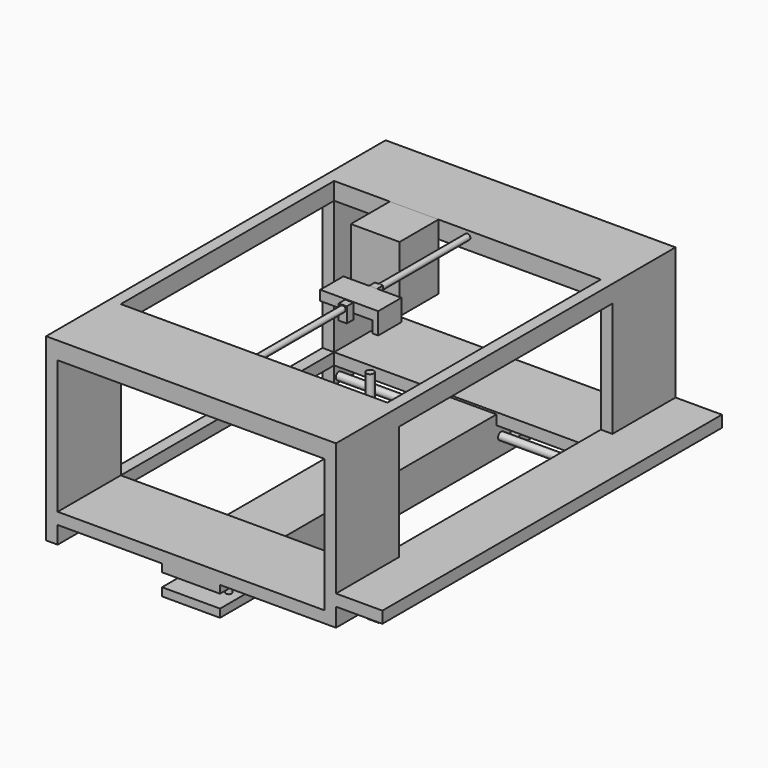
from build123d import *

# Parameters (mm, degrees)
F0_W         = 250
F0_H         = 250
F1_DEPTH     = 70
F2_T         = -10
F3_W         = 230
F3_H         = 120
F4_DEPTH     = 300
F5_W         = 230
F5_H         = 120
F6_DEPTH     = 300
F7_W         = 230
F7_H         = 230
F8_DEPTH     = 500
F9_W         = 10
F9_H         = 10
F1_FACE3_W   = 250
F1_FACE3_H   = 250
F1_FACE3_W_2 = 230
F1_FACE3_H_2 = 230
F10_DEPTH    = 15
F11_R        = 2.5
F12_DEPTH    = 250
F13_W        = 50
F13_H        = 18.5
F14_DEPTH    = 12.5
F16_DEPTH    = 10
F17_W        = 7
F17_H        = 13
F18_DEPTH    = 3.5
F19_R        = 3.25
F20_DEPTH    = 240
F21_W        = 50
F21_H        = 33.3125502616
F22_DEPTH    = 115
F23_R        = 3.25
F24_DEPTH    = 240
F25_R        = 3.25
F26_DEPTH    = 100
F27_W        = 42
F27_H        = 42
F28_DEPTH    = 56.5
F29_W        = 230
F29_H        = 115
F30_DEPTH    = 58
F31_W        = 230
F31_H        = 115
F32_DEPTH    = 58
F33_W        = 50
F33_H        = 25
F34_DEPTH    = 15
F35_W        = 50
F35_H        = 6.9269549847
F35_H_2      = 6.6508132219
F36_DEPTH    = 53
F37_R        = 2.5
F38_DEPTH    = 11.4222317934
F39_W        = 10
F39_H        = 230
F40_DEPTH    = 25
F41_W        = 40
F41_H        = 10
F41_W_2      = 10
F42_DEPTH    = 230
F43_W        = 40
F43_H        = 10
F44_DEPTH    = 68
F45_W        = 45.9353046417
F45_H        = 15
F46_DEPTH    = 25
F47_DEPTH    = 68
F48_W        = 45.9353
F48_H        = 15
F49_DEPTH    = 25
F50_DEPTH    = 68
F51_W        = 53
F51_H        = 11.3
F52_DEPTH    = 50
F53_R        = 2.5
F54_DEPTH    = 18.3


with BuildPart() as f1:
    # F0 (on Top) → F1 (new body, symmetric)
    with BuildSketch(Plane.XY):
        Rectangle(F0_W, F0_H)
    extrude(amount=F1_DEPTH, both=True)

    # F2
    f2_openings = [f1.faces().sort_by_distance(p)[0] for p in [
        (0, 0, 70),
    ]]
    offset(amount=F2_T, openings=f2_openings)

    # F3 (on face) → F4 (cut)
    with BuildSketch(Plane.XZ.offset(125)):
        Rectangle(F3_W, F3_H)
    extrude(amount=-F4_DEPTH, mode=Mode.SUBTRACT)

    # F5 (on face) → F6 (cut)
    with BuildSketch(Plane(origin=(-125, 0, 0), x_dir=(0, -1, 0), z_dir=(-1, 0, 0))):
        Rectangle(F5_W, F5_H)
    extrude(amount=-F6_DEPTH, mode=Mode.SUBTRACT)

    # F7 (on face) → F8 (cut)
    with BuildSketch(Plane.XY.offset(-60)):
        Rectangle(F7_W, F7_H)
    extrude(amount=-F8_DEPTH, mode=Mode.SUBTRACT)

    # F9 (on face) + F1_face3 (on face) → F10 (join)
    with BuildSketch(Plane(origin=(0, 0, -70), x_dir=(1, 0, 0), z_dir=(0, 0, -1))):
        with Locations((-120, -120)):
            Rectangle(F9_W, F9_H)
        with Locations((-120, 120)):
            Rectangle(F9_W, F9_H)
        with Locations((120, -120)):
            Rectangle(F9_W, F9_H)
        with Locations((120, 120)):
            Rectangle(F9_W, F9_H)
    with BuildSketch(Plane.XY.offset(70)):
        Rectangle(F1_FACE3_W, F1_FACE3_H)
        Rectangle(F1_FACE3_W_2, F1_FACE3_H_2, mode=Mode.SUBTRACT)
    extrude(amount=F10_DEPTH, dir=(0, 0, -1))

    # F11 (on face) → F12 (join)
    with BuildSketch(Plane(origin=(0, 125, 0), x_dir=(-1, 0, 0), z_dir=(0, 1, 0))):
        with Locations((0, 65)):
            Circle(F11_R)
    extrude(amount=-F12_DEPTH)

    # F13 (on Front) → F14 (join, symmetric)
    with BuildSketch(Plane.XZ):
        with Locations((0, 59.25)):
            Rectangle(F13_W, F13_H)
    extrude(amount=F14_DEPTH, both=True)

    # F15 (on face) → F16 (cut)
    with BuildSketch(Plane(origin=(0, 0, 50), x_dir=(1, 0, 0), z_dir=(0, 0, -1))):
        Polygon((20, -12.5), (20, 7.5), (20, 12.5), (-25, 12.5), (-25, -12.5), align=None)
    extrude(amount=-F16_DEPTH, mode=Mode.SUBTRACT)

    # F17 (on Right) → F18 (join, symmetric)
    with BuildSketch(Plane.YZ):
        with Locations((-16, 61.5)):
            Rectangle(F17_W, F17_H)
        with Locations((16, 61.5)):
            Rectangle(F17_W, F17_H)
    extrude(amount=F18_DEPTH, both=True)

    # F19 (on face) → F20 (join)
    with BuildSketch(Plane.YZ.offset(-115)):
        with Locations((120, -80)):
            Circle(F19_R)
    extrude(amount=F20_DEPTH)

    # F21 (on Front) → F22 (join, symmetric)
    with BuildSketch(Plane.XZ):
        with Locations((0, -78.3437248692)):
            Rectangle(F21_W, F21_H)
    extrude(amount=F22_DEPTH, both=True)

    # F23 (on face) → F24 (join)
    with BuildSketch(Plane(origin=(115, 0, 0), x_dir=(0, -1, 0), z_dir=(-1, 0, 0))):
        with Locations((120, -80)):
            Circle(F23_R)
    extrude(amount=F24_DEPTH)

    # F25 (on face) → F26 (join)
    with BuildSketch(Plane(origin=(0, 0, -95), x_dir=(1, 0, 0), z_dir=(0, 0, -1))):
        with Locations((0, -10)):
            Circle(F25_R)
    extrude(amount=-F26_DEPTH)

    # F29 (on face) → F30 (join)
    with BuildSketch(Plane(origin=(0, 125, 0), x_dir=(-1, 0, 0), z_dir=(0, 1, 0))):
        Polygon((-115, -85), (-115, -70), (115, -70), (115, -85), (125, -85), (125, 70), (-125, 70), (-125, -85), align=None)
        with Locations((0, -2.5)):
            Rectangle(F29_W, F29_H, mode=Mode.SUBTRACT)
    extrude(amount=F30_DEPTH)

    # F31 (on face) → F32 (join)
    with BuildSketch(Plane.XZ.offset(125)):
        Polygon((125, 70), (-125, 70), (-125, -85), (-115, -85), (-115, -70), (115, -70), (115, -85), (125, -85), align=None)
        with Locations((0, -2.5)):
            Rectangle(F31_W, F31_H, mode=Mode.SUBTRACT)
    extrude(amount=F32_DEPTH)

    # F33 (on face) → F34 (join)
    with BuildSketch(Plane(origin=(0, 115, 0), x_dir=(-1, 0, 0), z_dir=(0, 1, 0))):
        with Locations((0, -82.5)):
            Rectangle(F33_W, F33_H)
    extrude(amount=F34_DEPTH)

    # F35 (on face) → F36 (join, through all)
    with BuildSketch(Plane(origin=(0, 130, 0), x_dir=(-1, 0, 0), z_dir=(0, 1, 0))):
        with Locations((0, -91.5365225077)):
            Rectangle(F35_W, F35_H)
        with Locations((0, -73.325406611)):
            Rectangle(F35_W, F35_H_2)
    extrude(amount=F36_DEPTH)

    # F37 (on face) → F38 (join, through all)
    with BuildSketch(Plane(origin=(0, 0, -76.6508132219), x_dir=(1, 0, 0), z_dir=(0, 0, -1))):
        with Locations((-15, -161)):
            Circle(F37_R)
        with Locations((15, -161)):
            Circle(F37_R)
    extrude(amount=F38_DEPTH)

    # F39 (on face) → F40 (cut)
    with BuildSketch(Plane(origin=(0, 0, -70), x_dir=(1, 0, 0), z_dir=(0, 0, -1))):
        with Locations((120, 0)):
            Rectangle(F39_W, F39_H)
    extrude(amount=-F40_DEPTH, mode=Mode.SUBTRACT)

    # F41 (on face) → F42 (join, through all)
    with BuildSketch(Plane.XZ.offset(-115)):
        with Locations((145, -49)):
            Rectangle(F41_W, F41_H)
        with Locations((120, -49)):
            Rectangle(F41_W_2, F41_H)
    extrude(amount=F42_DEPTH)

    # F43 (on face) → F44 (join, through all)
    with BuildSketch(Plane(origin=(0, 115, 0), x_dir=(-1, 0, 0), z_dir=(0, 1, 0))):
        with Locations((-145, -49)):
            Rectangle(F43_W, F43_H)
    extrude(amount=F44_DEPTH)

    # F45 (on face) → F46 (cut)
    with BuildSketch(Plane(origin=(115, 0, 0), x_dir=(0, -1, 0), z_dir=(-1, 0, 0))):
        with Locations((-160.0323476791, -77.5)):
            Rectangle(F45_W, F45_H)
    extrude(amount=-F46_DEPTH, mode=Mode.SUBTRACT)

    # F47 (add, through all): a face of the model
    f47_faces = [f1.faces().sort_by_distance(p)[0] for p in [
        (145, -115, -49),
    ]]
    extrude(f47_faces, amount=F47_DEPTH)

    # F48 (on face) → F49 (cut)
    with BuildSketch(Plane.YZ.offset(125)):
        with Locations((-160.03235, -77.5)):
            Rectangle(F48_W, F48_H)
    extrude(amount=-F49_DEPTH, mode=Mode.SUBTRACT)

    # F50 (add, through all): a face of the model
    f50_faces = [f1.faces().sort_by_distance(p)[0] for p in [
        (0, -115, -82.5),
    ]]
    extrude(f50_faces, amount=F50_DEPTH)

    # F51 (on face) → F52 (cut)
    with BuildSketch(Plane.YZ.offset(25)):
        with Locations((-156.5, -82.35)):
            Rectangle(F51_W, F51_H)
    extrude(amount=-F52_DEPTH, mode=Mode.SUBTRACT)

    # F53 (on face) → F54 (join, through all)
    with BuildSketch(Plane(origin=(0, 0, -76.7), x_dir=(1, 0, 0), z_dir=(0, 0, -1))):
        with Locations((15, 161)):
            Circle(F53_R)
        with Locations((-15, 161)):
            Circle(F53_R)
    extrude(amount=F54_DEPTH)


with BuildPart() as f28:
    # F27 (on face) → F28 (new body)
    with BuildSketch(Plane.XY.offset(70)):
        with Locations((-46, 94)):
            Rectangle(F27_W, F27_H)
    extrude(amount=-F28_DEPTH)


solid = Compound([f1.part, f28.part])
